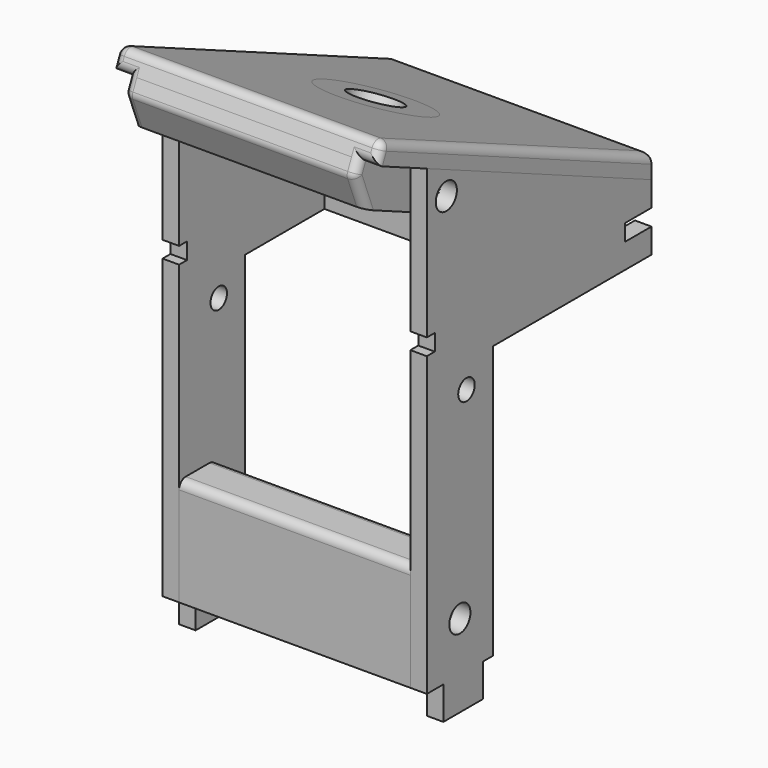
from build123d import *

# Parameters (mm, degrees)
F0_R           = 1.6
F0_R_2         = 1.25
F1_DEPTH       = 2
F4_W           = 28
F4_H           = 12
F5_DEPTH       = 3
F6_W           = 28
F6_H           = 8
F7_DEPTH       = 2
F9_W           = 28
F9_H           = 13
F10_DEPTH      = 10
F11_R          = 1.6
F12_DEPTH      = 28
F13_DEPTH      = 30
F13_DEPTH_BACK = 2
F14_SIZE       = 3
F15_T1_DEPTH   = 4.000001254
F15_T3_DEPTH   = 1.4294797395
F15_T5_DEPTH   = 45.9213150338
F15_T7_DEPTH   = 26
F15_T9_DEPTH   = 6.3284271247
F15_T11_DEPTH  = 30
F15_T13_DEPTH  = 4.5000031963
F15_T15_DEPTH  = 4.5000031963
F15_T17_DEPTH  = 35.2590858648
F15_T22_DEPTH  = 1
F15_T28_DEPTH  = 1
F15_T34_DEPTH  = 1
F15_T40_DEPTH  = 1
F15_T47_DEPTH  = 3.9294797395
F15_T51_DEPTH  = 7.0000063926
F15_T58_DEPTH  = 3.9294797395
F15_T62_DEPTH  = 7.0000063926
F15_2_T1_DEPTH = 33
F16_R          = 6.25
F16_R_2        = 3
F17_DEPTH      = 10
F18_DEPTH      = 2.5
F19_R          = 1
F20_SIZE2      = 1.5
F20_SIZE       = 4
F21_DEPTH      = 28
F22_SIZE       = 5
F23_R          = 1


# Not quite as in the source:
# - a fillet or chamfer that OpenCascade refuses, or shapes differently, is made with other operations: its cross-section is extruded or revolved along the edge and cut away or added
# - a feature names something its author has since deleted; it is built from what else it names


with BuildPart() as f1:
    # F0 (on Right) → F1 (new body)
    with BuildSketch(Plane.YZ):
        Polygon((-17, 37), (-17, 22), (17, 22), align=None)
        with Locations((-14.0519337729, 32.868342638)):
            Circle(F0_R, mode=Mode.SUBTRACT)
        Polygon((-14.5, -19), (-14.5, -23), (-8.5, -23), (-8.5, -19), (-7, -19), (-7, 14), (17, 14), (17, 17), (13, 17), (13, 19), (17, 19), (17, 22), (-17, 22), (-17, 19), (-15.8, 19), (-15.8, 17), (-17, 17), (-17, -19), align=None)
        with Locations((-12, -13)):
            Circle(F0_R, mode=Mode.SUBTRACT)
        with Locations((-11, 11)):
            Circle(F0_R_2, mode=Mode.SUBTRACT)
    extrude(amount=F1_DEPTH)


with BuildPart() as f3_1:
    # F3: copy of F1
    add(f1.part.moved(Location((-30, 0, 0))))


with BuildPart() as f5:
    # F4 (on face) → F5 (new body)
    with BuildSketch(Plane(origin=(0, 0, 14), x_dir=(1, 0, 0), z_dir=(0, 0, -1))):
        with Locations((-14, -11)):
            Rectangle(F4_W, F4_H)
    extrude(amount=-F5_DEPTH)


with BuildPart() as f7:
    # F6 (on face) → F7 (new body)
    with BuildSketch(Plane.XY.offset(17)):
        with Locations((-14.0000008643, 9)):
            Rectangle(F6_W, F6_H)
    extrude(amount=F7_DEPTH)


with BuildPart() as f8_1:
    # F8: copy of F5
    add(f5.part.moved(Location((0, 0, 5))))


with BuildPart() as f10:
    # F9 (on face) → F10 (new body)
    with BuildSketch(Plane.XZ.offset(17)):
        with Locations((-14, -12.5)):
            Rectangle(F9_W, F9_H)
    extrude(amount=-F10_DEPTH)

    # F15#2: fillet of radius 1 on 1 edges, made by hand

    # F15_2_s2 → F15_2_t1 (cut)
    with BuildSketch(Plane.YZ.offset(-30.5)):
        with BuildLine():
            ThreePointArc((-16, -6), (-16.7071067812, -6.2928932188), (-17, -7))
            Line((-17, -7), (-17, -6))
            Line((-17, -6), (-16, -6))
        make_face()
    extrude(amount=F15_2_T1_DEPTH, mode=Mode.SUBTRACT)

    # F0 (on Right) → F21 (cut)
    with BuildSketch(Plane.YZ):
        with Locations((-12, -13)):
            Circle(F0_R)
    extrude(amount=-F21_DEPTH, mode=Mode.SUBTRACT)

    # F22
    f22_edges = [f10.edges().sort_by_distance(p)[0] for p in [
        (-14, -7, -6),
    ]]
    chamfer(f22_edges, length=F22_SIZE)

    # F23
    f23_edges = [f10.edges().sort_by_distance(p)[0] for p in [
        (-14, -12, -6),
        (-14, -7, -11),
    ]]
    fillet(f23_edges, radius=F23_R)


with BuildPart() as f12:
    # F11 (on Right) → F12 (new body)
    with BuildSketch(Plane.YZ):
        Polygon((5, 22), (17, 22), (-24.6509383276, 40.3754630187), (-26.6060520612, 35.9438837188), align=None)
        with Locations((-14.0607692301, 32.8608974814)):
            Circle(F11_R, mode=Mode.SUBTRACT)
    extrude(amount=-F12_DEPTH)

    # F11 (on Right) → F13 (join, two sides)
    with BuildSketch(Plane.YZ) as f13_sk:
        Polygon((-24.6509383276, 40.3754630187), (17, 22), (17, 24.7324859082), (-23.641832632, 42.6627552377), align=None)
    extrude(amount=-F13_DEPTH)
    extrude(f13_sk.sketch, amount=F13_DEPTH_BACK)

    # F14
    f14_edges = [f12.edges().sort_by_distance(p)[0] for p in [
        (-14, -26.606052, 35.943884),
    ]]
    chamfer(f14_edges, length=F14_SIZE)

    # F15: fillet of radius 1 on 14 edges, made by hand

    # F15_s2 → F15_t1 (cut)
    with BuildSketch(Plane(origin=(0, 11.4997819512, 26.0660126014), x_dir=(1, 0, 0), z_dir=(0, -0.4036422782, -0.9149168876))):
        with BuildLine():
            ThreePointArc((-29, 38.8508036488), (-29.7071067812, 38.55791043), (-30, 37.8508036488))
            Line((-30, 37.8508036488), (-30, 38.8508036488))
            Line((-30, 38.8508036488), (-29, 38.8508036488))
        make_face()
        with BuildLine():
            ThreePointArc((1, 38.8508036488), (1.7071067812, 38.55791043), (2, 37.8508036488))
            Line((2, 37.8508036488), (2, 38.8508036488))
            Line((2, 38.8508036488), (1, 38.8508036488))
        make_face()
    extrude(amount=F15_T1_DEPTH, mode=Mode.SUBTRACT)

    # F15_s4 → F15_t3 (cut)
    with BuildSketch(Plane(origin=(0, 10.8943065058, 24.6936954967), x_dir=(1, 0, 0), z_dir=(0, -0.4036411085, -0.9149174037))):
        with BuildLine():
            ThreePointArc((-27, 38.8507691414), (-27.7071067812, 38.5578759226), (-28, 37.8507691414))
            Line((-28, 37.8507691414), (-28, 38.8507691414))
            Line((-28, 38.8507691414), (-27, 38.8507691414))
        make_face()
        with BuildLine():
            ThreePointArc((-1, 38.8507691414), (-0.2928932188, 38.5578759226), (0, 37.8507691414))
            Line((0, 37.8507691414), (0, 38.8507691414))
            Line((0, 38.8507691414), (-1, 38.8507691414))
        make_face()
    extrude(amount=F15_T3_DEPTH, mode=Mode.SUBTRACT)

    # F15_s6 → F15_t5 (cut)
    with BuildSketch(Plane(origin=(0, 7.3838839309, -3.2576047635), x_dir=(1, 0, 0), z_dir=(0, -0.9149173938, 0.4036411309))):
        with BuildLine():
            ThreePointArc((1, 29.4900807741), (1.7071067812, 29.1971875553), (2, 28.4900807741))
            Line((2, 28.4900807741), (2, 29.4900807741))
            Line((2, 29.4900807741), (1, 29.4900807741))
        make_face()
        with BuildLine():
            ThreePointArc((-29, 29.4900807741), (-29.7071067812, 29.1971875553), (-30, 28.4900807741))
            Line((-30, 28.4900807741), (-30, 29.4900807741))
            Line((-30, 29.4900807741), (-29, 29.4900807741))
        make_face()
    extrude(amount=F15_T5_DEPTH, mode=Mode.SUBTRACT)

    # F15_s8 → F15_t7 (cut)
    with BuildSketch(Plane.YZ.offset(-27)):
        with BuildLine():
            ThreePointArc((-25.2279351142, 39.0676071268), (-25.3127579386, 38.6867580446), (-25.2453793759, 38.3024390829))
            Line((-25.2453793759, 38.3024390829), (-25.3951287357, 38.6886359298))
            Line((-25.3951287357, 38.6886359298), (-25.2279351142, 39.0676071268))
        make_face()
    extrude(amount=F15_T7_DEPTH, mode=Mode.SUBTRACT)

    # F15_s10 → F15_t9 (cut)
    with BuildSketch(Plane(origin=(0, -16.2103654509, 41.8058015836), x_dir=(1, 0, 0), z_dir=(0, 0.3615269354, -0.9323616653))):
        with BuildLine():
            ThreePointArc((0, 8.6904605378), (-0.2928932188, 9.397567319), (-1, 9.6904605378))
            Line((-1, 9.6904605378), (0, 9.6904605378))
            Line((0, 9.6904605378), (0, 8.6904605378))
        make_face()
        with BuildLine():
            ThreePointArc((-27, 9.6904605378), (-27.7071067812, 9.397567319), (-28, 8.6904605378))
            Line((-28, 8.6904605378), (-28, 9.6904605378))
            Line((-28, 9.6904605378), (-27, 9.6904605378))
        make_face()
    extrude(amount=F15_T9_DEPTH, mode=Mode.SUBTRACT)

    # F15_s12 → F15_t11 (cut)
    with BuildSketch(Plane.YZ.offset(-29)):
        with BuildLine():
            ThreePointArc((-24.0454744041, 41.7478394975), (-23.4920838444, 42.2765591201), (-22.7269163856, 42.259114613))
            Line((-22.7269163856, 42.259114613), (-23.641832632, 42.6627552377))
            Line((-23.641832632, 42.6627552377), (-24.0454744041, 41.7478394975))
        make_face()
    extrude(amount=F15_T11_DEPTH, mode=Mode.SUBTRACT)

    # F15_s14 → F15_t13 (cut)
    with BuildSketch(Plane.YZ.offset(-32.5000031963)):
        with BuildLine():
            ThreePointArc((-24.2472955333, 41.290381076), (-24.2647405421, 40.5252124585), (-23.7360197542, 39.9718213941))
            Line((-23.7360197542, 39.9718213941), (-24.6509383276, 40.3754630187))
            Line((-24.6509383276, 40.3754630187), (-24.2472955333, 41.290381076))
        make_face()
    extrude(amount=F15_T13_DEPTH, mode=Mode.SUBTRACT)

    # F15_s16 → F15_t15 (cut)
    with BuildSketch(Plane.YZ):
        with BuildLine():
            ThreePointArc((-24.2472955333, 41.290381076), (-24.2647405421, 40.5252124585), (-23.7360197542, 39.9718213941))
            Line((-23.7360197542, 39.9718213941), (-24.6509383276, 40.3754630187))
            Line((-24.6509383276, 40.3754630187), (-24.2472955333, 41.290381076))
        make_face()
    extrude(amount=F15_T15_DEPTH, mode=Mode.SUBTRACT)

    # F15_s18 → F15_t17 (cut)
    with BuildSketch(Plane.YZ.offset(-31.6295429324)):
        with BuildLine():
            ThreePointArc((16.4036411309, 24.9955861291), (16.837747316, 24.6267268224), (17, 24.0806687353))
            Line((17, 24.0806687353), (17, 24.7324859082))
            Line((17, 24.7324859082), (16.4036411309, 24.9955861291))
        make_face()
    extrude(amount=F15_T17_DEPTH, mode=Mode.SUBTRACT)


with BuildPart() as f15_tool20:
    # F15_s21 → F15_t22 (new body)
    with BuildSketch(Plane.YZ.offset(-29)):
        Polygon((-23.1305575165, 41.3441972192), (-24.0454744041, 41.7478394975), (-23.641832632, 42.6627552377), (-22.7269163856, 42.259114613), align=None)
    extrude(amount=-F15_T22_DEPTH)

    # F15_s23 → F15_t24 (revolve, cut)
    with BuildSketch(Plane(origin=(-29, -23.1305575165, 41.3441972192), x_dir=(0, 0.3615263279, -0.9323619009), z_dir=(0, 0.9323619009, 0.3615263279))):
        with BuildLine():
            ThreePointArc((0, -1), (1, 0), (0, 1))
            Line((0, 1), (0, -1))
        make_face()
    revolve(axis=Axis((-29, -23.1305575165, 41.3441972192), (-1, 0, 0)), mode=Mode.SUBTRACT)


with BuildPart() as f12_1:
    add(f12.part)

    # F15_t19: cut F15_tool20
    add(f15_tool20.part, mode=Mode.SUBTRACT)


with BuildPart() as f15_tool26:
    # F15_s27 → F15_t28 (new body)
    with BuildSketch(Plane.YZ.offset(1)):
        Polygon((-23.1305575165, 41.3441972192), (-22.7269163856, 42.259114613), (-23.641832632, 42.6627552377), (-24.0454744041, 41.7478394975), align=None)
    extrude(amount=F15_T28_DEPTH)

    # F15_s29 → F15_t30 (revolve, cut)
    with BuildSketch(Plane(origin=(1, -23.1305575165, 41.3441972192), x_dir=(0, 0.3615263279, -0.9323619009), z_dir=(0, -0.9323619009, -0.3615263279))):
        with BuildLine():
            ThreePointArc((0, -1), (1, 0), (0, 1))
            Line((0, 1), (0, -1))
        make_face()
    revolve(axis=Axis((1, -23.1305575165, 41.3441972192), (1, 0, 0)), mode=Mode.SUBTRACT)


with BuildPart() as f12_2:
    add(f12_1.part)

    # F15_t25: cut F15_tool26
    add(f15_tool26.part, mode=Mode.SUBTRACT)


with BuildPart() as f15_tool32:
    # F15_s33 → F15_t34 (new body)
    with BuildSketch(Plane.YZ.offset(-27)):
        Polygon((-24.3130177106, 38.6639660183), (-25.2279351142, 39.0676071268), (-25.3951287357, 38.6886359298), (-25.2453793759, 38.3024390829), align=None)
    extrude(amount=-F15_T34_DEPTH)

    # F15_s35 → F15_t36 (revolve, cut)
    with BuildSketch(Plane(origin=(-27, -24.3130177106, 38.6639660183), x_dir=(0, 0.999740228, -0.0227920262), z_dir=(0, 0.0227920262, 0.999740228))):
        with BuildLine():
            ThreePointArc((0, -1), (1, 0), (0, 1))
            Line((0, 1), (0, -1))
        make_face()
    revolve(axis=Axis((-27, -24.3130177106, 38.6639660183), (-1, 0, 0)), mode=Mode.SUBTRACT)


with BuildPart() as f12_3:
    add(f12_2.part)

    # F15_t31: cut F15_tool32
    add(f15_tool32.part, mode=Mode.SUBTRACT)


with BuildPart() as f15_tool38:
    # F15_s39 → F15_t40 (new body)
    with BuildSketch(Plane.YZ.offset(-1)):
        Polygon((-24.3130177106, 38.6639660183), (-25.2453793759, 38.3024390829), (-25.3951287357, 38.6886359298), (-25.2279351142, 39.0676071268), align=None)
    extrude(amount=F15_T40_DEPTH)

    # F15_s41 → F15_t42 (revolve, cut)
    with BuildSketch(Plane(origin=(-1, -24.3130177106, 38.6639660183), x_dir=(0, 0.999740228, -0.0227920262), z_dir=(0, -0.0227920262, -0.999740228))):
        with BuildLine():
            ThreePointArc((0, -1), (1, 0), (0, 1))
            Line((0, 1), (0, -1))
        make_face()
    revolve(axis=Axis((-1, -24.3130177106, 38.6639660183), (1, 0, 0)), mode=Mode.SUBTRACT)


with BuildPart() as f12_4:
    add(f12_3.part)

    # F15_t37: cut F15_tool38
    add(f15_tool38.part, mode=Mode.SUBTRACT)


with BuildPart() as f15_tool45:
    # F15_s46 → F15_t47 (new body)
    with BuildSketch(Plane(origin=(0, 11.903409277, 26.9809890059), x_dir=(1, 0, 0), z_dir=(0, -0.4036411085, -0.9149174037))):
        with BuildLine():
            ThreePointArc((-27, 38.8507691414), (-27.7071067812, 38.5578759226), (-28, 37.8507691414))
            Line((-28, 37.8507691414), (-28, 38.8507691414))
            Line((-28, 38.8507691414), (-27, 38.8507691414))
        make_face()
    extrude(amount=F15_T47_DEPTH)

    split(bisect_by=Plane(origin=(0, 10.8943065058, 24.6936954967), x_dir=(1, 0, 0), z_dir=(0, 0.4036411085, 0.9149174037)), keep=Keep.TOP)


with BuildPart() as f15_tool49:
    # F15_s50 → F15_t51 (new body)
    with BuildSketch(Plane.YZ.offset(-32.5000031963)):
        with BuildLine():
            ThreePointArc((-24.2472955333, 41.290381076), (-24.2647405421, 40.5252124585), (-23.7360197542, 39.9718213941))
            Line((-23.7360197542, 39.9718213941), (-24.6509383276, 40.3754630187))
            Line((-24.6509383276, 40.3754630187), (-24.2472955333, 41.290381076))
        make_face()
    extrude(amount=F15_T51_DEPTH)

    split(bisect_by=Plane.YZ.offset(-28), keep=Keep.TOP)


with BuildPart() as f15_tool45_1:
    add(f15_tool45.part)

    # F15_t53: intersect F15_tool49
    add(f15_tool49.part, mode=Mode.INTERSECT)


with BuildPart() as f12_5:
    add(f12_4.part)

    # F15_t43: cut F15_tool45
    add(f15_tool45_1.part, mode=Mode.SUBTRACT)


with BuildPart() as f15_tool56:
    # F15_s57 → F15_t58 (new body)
    with BuildSketch(Plane(origin=(0, 11.903409277, 26.9809890059), x_dir=(1, 0, 0), z_dir=(0, -0.4036411085, -0.9149174037))):
        with BuildLine():
            ThreePointArc((-1, 38.8507691414), (-0.2928932188, 38.5578759226), (0, 37.8507691414))
            Line((0, 37.8507691414), (0, 38.8507691414))
            Line((0, 38.8507691414), (-1, 38.8507691414))
        make_face()
    extrude(amount=F15_T58_DEPTH)

    split(bisect_by=Plane(origin=(0, 10.8943065058, 24.6936954967), x_dir=(1, 0, 0), z_dir=(0, 0.4036411085, 0.9149174037)), keep=Keep.TOP)


with BuildPart() as f15_tool60:
    # F15_s61 → F15_t62 (new body)
    with BuildSketch(Plane.YZ.offset(-2.5000031963)):
        with BuildLine():
            ThreePointArc((-24.2472955333, 41.290381076), (-24.2647405421, 40.5252124585), (-23.7360197542, 39.9718213941))
            Line((-23.7360197542, 39.9718213941), (-24.6509383276, 40.3754630187))
            Line((-24.6509383276, 40.3754630187), (-24.2472955333, 41.290381076))
        make_face()
    extrude(amount=F15_T62_DEPTH)

    split(bisect_by=Plane.YZ, keep=Keep.BOTTOM)


with BuildPart() as f15_tool56_1:
    add(f15_tool56.part)

    # F15_t64: intersect F15_tool60
    add(f15_tool60.part, mode=Mode.INTERSECT)


with BuildPart() as f12_6:
    add(f12_5.part)

    # F15_t54: cut F15_tool56
    add(f15_tool56_1.part, mode=Mode.SUBTRACT)

    # F16 (on face) → F17 (cut)
    with BuildSketch(Plane(origin=(0, 11.9034095536, 26.9809878445), x_dir=(1, 0, 0), z_dir=(0, 0.4036411309, 0.9149173938))):
        with Locations((-14, -18.198827429)):
            Circle(F16_R)
        with Locations((-14, -18.198827429)):
            Circle(F16_R_2, mode=Mode.SUBTRACT)
        with Locations((-14, -18.198827429)):
            Circle(F16_R_2)
    extrude(amount=-F17_DEPTH, mode=Mode.SUBTRACT)

    # F16 (on face) → F18 (join)
    with BuildSketch(Plane(origin=(0, 11.9034095536, 26.9809878445), x_dir=(1, 0, 0), z_dir=(0, 0.4036411309, 0.9149173938))):
        with Locations((-14, -18.198827429)):
            Circle(F16_R)
        with Locations((-14, -18.198827429)):
            Circle(F16_R_2, mode=Mode.SUBTRACT)
    extrude(amount=-F18_DEPTH)

    # F19
    f19_edges = [f12_6.edges().sort_by_distance(p)[0] for p in [
        (-20.25, -7.711231, 27.607911),
    ]]
    fillet(f19_edges, radius=F19_R)


with BuildPart() as f5_1:
    add(f5.part)

    # F20
    f20_edges = [f5_1.edges().sort_by_distance(p)[0] for p in [
        (-14, 17, 17),
    ]]
    f20_side = f5_1.faces().sort_by_distance((-14, 11, 17))[0]
    chamfer(f20_edges, length=F20_SIZE, length2=F20_SIZE2, reference=f20_side)


solid = Compound([f1.part, f3_1.part, f7.part, f8_1.part, f10.part, f12_6.part, f5_1.part])
